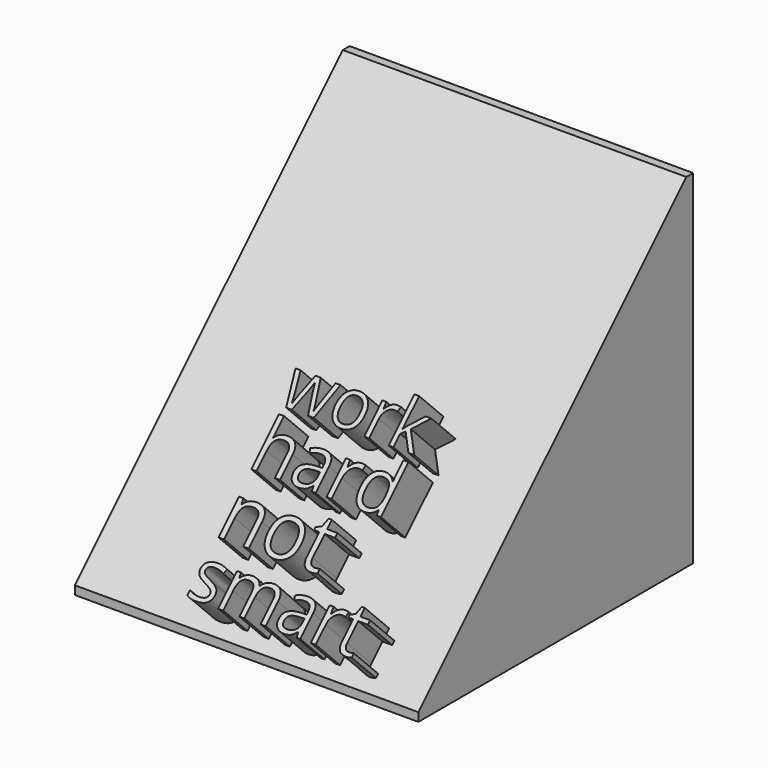
from build123d import *

# Parameters (mm, degrees)
F0_W           = 50.8
F0_H           = 50.8
F1_DEPTH       = 50.8
F2_SIZE        = 49.53
F3_TEXT_SIZE   = 8.8194444444
F3_TEXT_SIZE_2 = 9.4978662991
F3_TEXT_SIZE_3 = 9.977233029
F3_TEXT_SIZE_4 = 9.2071114232
F4_DEPTH       = 6.35


# Not quite as in the source:
# - Text() gives the source's letters only with a copy of the font that has no kerning and outlines rounded to 1/6400 em; it was checked with that copy


with BuildPart() as f1:
    # F0 (on Top) → F1 (new body)
    with BuildSketch(Plane.XY):
        with Locations((3.07e-07, 0.0025036842)):
            Rectangle(F0_W, F0_H)
    extrude(amount=F1_DEPTH)

    # F2
    f2_edges = [f1.edges().sort_by_distance(p)[0] for p in [
        (0, -25.397496, 50.8),
    ]]
    chamfer(f2_edges, length=F2_SIZE)

    # F3 (on face) → F4 (join)
    with BuildSketch(Plane(origin=(0, -13.3337481579, 13.3337481579), x_dir=(1, 0, 0), z_dir=(0, -0.7071067812, 0.7071067812))):
        with Locations((-7.1990872504, 9.9125494308)):
            Text('work', F3_TEXT_SIZE, font='Open Sans', text_align=(TextAlign.LEFT, TextAlign.BOTTOM))
        with Locations((-7.1293068904, 1.6784803182)):
            Text('hard', F3_TEXT_SIZE_2, font='Open Sans', text_align=(TextAlign.LEFT, TextAlign.BOTTOM))
        with Locations((-6.9897467781, -7.1836077808)):
            Text('not', F3_TEXT_SIZE_3, font='Open Sans', text_align=(TextAlign.LEFT, TextAlign.BOTTOM))
        with Locations((-6.9199664181, -15.0687720551)):
            Text('smart', F3_TEXT_SIZE_4, font='Open Sans', text_align=(TextAlign.LEFT, TextAlign.BOTTOM))
    extrude(amount=F4_DEPTH)


solid = f1.part
